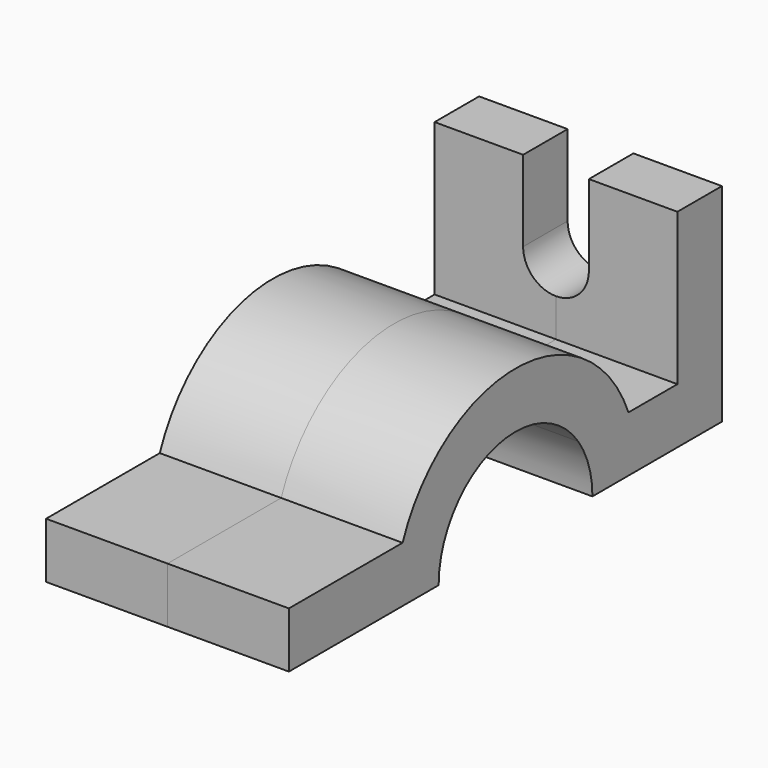
from build123d import *

# Parameters (mm, degrees)
F0_W     = 11
F0_H     = 30
F1_DEPTH = 24
F3_DEPTH = 11


# Not quite as in the source:
# - a feature of the source that left no trace in its solid (it failed there, or was rolled back) is left out


with BuildPart() as f1:
    # F0 (on Right) → F1 (new body, symmetric)
    with BuildSketch(Plane.YZ):
        with BuildLine():
            ThreePointArc((15.4919333848, 11), (18.1017503893, 5.7729223833), (19, 0))
            Line((19, 0), (30, 0))
            ThreePointArc((30, 0), (29.4730143031, 5.5983415304), (27.9105714739, 11))
            Line((27.9105714739, 11), (15.4919333848, 11))
        make_face()
        with BuildLine():
            ThreePointArc((-15.4919333848, 11), (0, 19), (15.4919333848, 11))
            Line((15.4919333848, 11), (27.9105714739, 11))
            ThreePointArc((27.9105714739, 11), (0, 30), (-27.9105714739, 11))
            Line((-27.9105714739, 11), (-15.4919333848, 11))
        make_face()
        with BuildLine():
            Line((-30, 0), (-19, 0))
            ThreePointArc((-19, 0), (-18.1017503893, 5.7729223833), (-15.4919333848, 11))
            Line((-15.4919333848, 11), (-27.9105714739, 11))
            ThreePointArc((-27.9105714739, 11), (-29.4730143031, 5.5983415304), (-30, 0))
        make_face()
        with BuildLine():
            ThreePointArc((27.9105714739, 11), (29.4730143031, 5.5983415304), (30, 0))
            Line((30, 0), (51, 0))
            Line((51, 0), (51, 11))
            Line((51, 11), (40, 11))
            Line((40, 11), (27.9105714739, 11))
        make_face()
        with BuildLine():
            Line((-56, 0), (-30, 0))
            ThreePointArc((-30, 0), (-29.4730143031, 5.5983415304), (-27.9105714739, 11))
            Line((-27.9105714739, 11), (-56, 11))
            Line((-56, 11), (-56, 0))
        make_face()
        with Locations((45.5, 26)):
            Rectangle(F0_W, F0_H)
    extrude(amount=F1_DEPTH, both=True)

    # F2 (on face) → F3 (cut, through all)
    with BuildSketch(Plane(origin=(0, 51, 0), x_dir=(-1, 0, 0), z_dir=(0, 1, 0))):
        with BuildLine():
            ThreePointArc((-6.5, 25), (0, 18.5), (6.5, 25))
            ThreePointArc((6.5, 25), (0, 31.5), (-6.5, 25))
        make_face()
        with BuildLine():
            ThreePointArc((-6.5, 25), (0, 31.5), (6.5, 25))
            Line((6.5, 25), (6.5, 41))
            Line((6.5, 41), (-6.5, 41))
            Line((-6.5, 41), (-6.5, 25))
        make_face()
    extrude(amount=-F3_DEPTH, mode=Mode.SUBTRACT)


solid = f1.part
